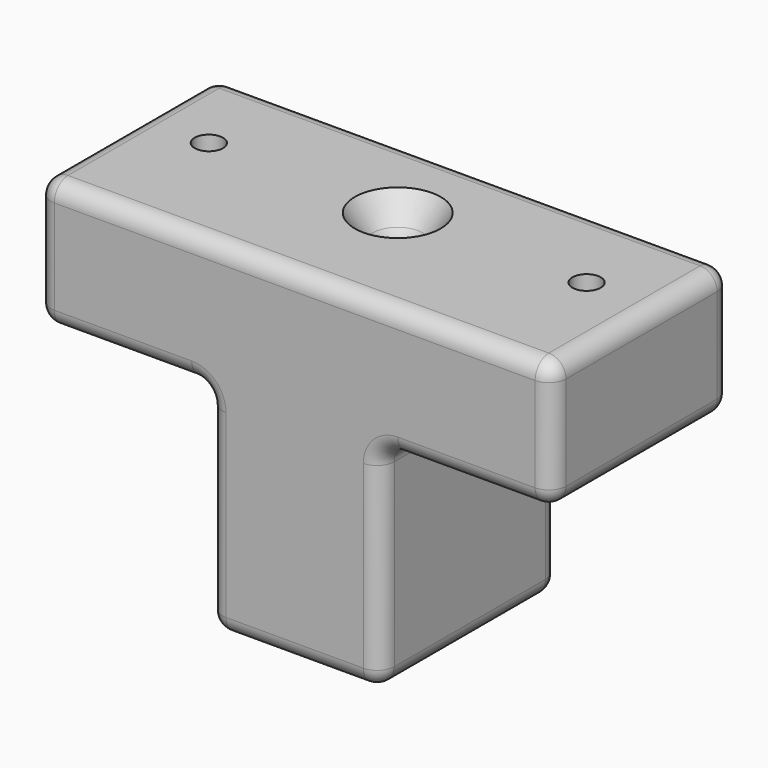
from build123d import *

# Parameters (mm, degrees)
F0_W      = 60
F0_H      = 26
F1_DEPTH  = 40
F5_R      = 2
F6_DEPTH  = 13
F8_D      = 3.3
F8_DEPTH  = 9
F8_TIP    = 0.9914200214
F9_R      = 4.3298566402
F10_DEPTH = 6
F11_W     = 20
F11_H     = 26
F12_DEPTH = 25
F13_R     = 2


with BuildPart() as f1:
    # F0 (on Top) → F1 (new body)
    with BuildSketch(Plane.XY):
        with Locations((30, 13)):
            Rectangle(F0_W, F0_H)
    extrude(amount=F1_DEPTH)

    # F3 (on offset) → F4 (revolve, cut)
    with BuildSketch(Plane.XZ.offset(-15)):
        with BuildLine():
            Line((35, 40), (30, 40))
            Line((30, 40), (30, 5))
            Line((30, 5), (32, 5))
            Line((32, 5), (32, 34.1348334202))
            ThreePointArc((32, 34.1348334202), (32.2309171832, 35.6367818503), (32.9023396346, 37))
            Line((32.9023396346, 37), (35, 40))
        make_face()
    revolve(axis=Axis((30, 15, 22.5), (0, 0, -1)), mode=Mode.SUBTRACT)

    # F5 (on face) → F6 (cut)
    with BuildSketch(Plane(origin=(0, 26, 0), x_dir=(-1, 0, 0), z_dir=(0, 1, 0))):
        with Locations((-30, 7)):
            Circle(F5_R)
    extrude(amount=-F6_DEPTH, mode=Mode.SUBTRACT)

    # F8
    with Locations(Plane.XY.offset(40)):
        with Locations((8, 15), (52, 15)):
            Hole(F8_D / 2, depth=F8_DEPTH)
            with Locations((0, 0, -(F8_DEPTH + F8_TIP / 2))):  # 118° drill point
                Cone(0, F8_D / 2, F8_TIP, mode=Mode.SUBTRACT)

    # F9 (on face) → F10 (cut)
    with BuildSketch(Plane(origin=(0, 26, 0), x_dir=(-1, 0, 0), z_dir=(0, 1, 0))):
        with Locations((-30, 7)):
            Circle(F9_R)
    extrude(amount=-F10_DEPTH, mode=Mode.SUBTRACT)

    # F11 (on face) → F12 (cut)
    with BuildSketch(Plane(origin=(0, 0, 0), x_dir=(1, 0, 0), z_dir=(0, 0, -1))):
        with Locations((10, -13)):
            Rectangle(F11_W, F11_H)
        with Locations((50, -13)):
            Rectangle(F11_W, F11_H)
    extrude(amount=-F12_DEPTH, mode=Mode.SUBTRACT)

    # F13
    f13_edges = [f1.edges().sort_by_distance(p)[0] for p in [
        (30, 26, 40),
        (30, 0, 40),
        (60, 13, 40),
        (0, 13, 40),
        (0, 0, 32.5),
        (10, 0, 25),
        (0, 13, 25),
        (20, 0, 12.5),
        (20, 13, 25),
        (20, 26, 12.5),
        (20, 13, 0),
        (30, 26, 0),
        (30, 0, 0),
        (40, 13, 0),
        (40, 26, 12.5),
        (40, 13, 25),
        (50, 26, 25),
        (60, 13, 25),
        (50, 0, 25),
        (40, 0, 12.5),
        (60, 26, 32.5),
        (60, 0, 32.5),
        (0, 26, 32.5),
        (10, 26, 25),
    ]]
    fillet(f13_edges, radius=F13_R)


solid = f1.part
